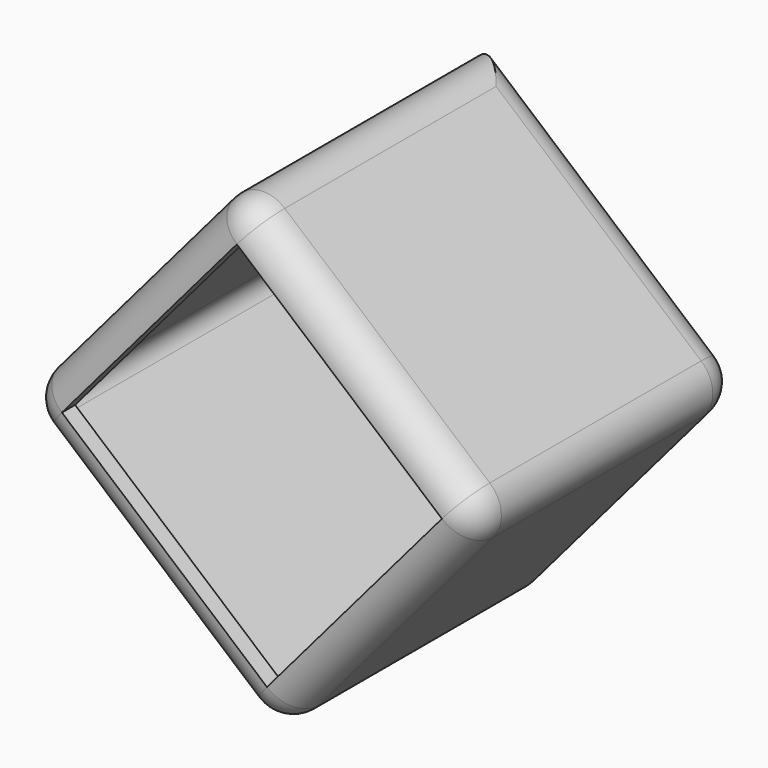
from build123d import *

# Parameters (mm, degrees)
F1_DEPTH = 50.8
F2_R     = 5.08
F3_T     = -2.54


# Not quite as in the source:
# - a shell that OpenCascade refuses in one call is made with other operations: the cavity is built on its own and cut out


with BuildPart() as f1:
    # F0 (on Front) → F1 (new body)
    with BuildSketch(Plane.XZ):
        Polygon((-36.388931796, -2.8822999448), (2.8822999448, -36.388931796), (36.388931796, 2.8822999448), (-2.8822999448, 36.388931796), align=None)
    extrude(amount=F1_DEPTH)

    # F2
    f2_edges = [f1.edges().sort_by_distance(p)[0] for p in [
        (36.388932, -25.4, 2.8823),
        (-2.8823, -25.4, 36.388932),
        (16.753316, 0, 19.635616),
        (16.753316, -50.8, 19.635616),
        (-19.635616, -50.8, 16.753316),
        (-16.753316, -50.8, -19.635616),
        (19.635616, -50.8, -16.753316),
        (2.8823, -25.4, -36.388932),
        (19.635616, 0, -16.753316),
        (-36.388932, -25.4, -2.8823),
        (-16.753316, 0, -19.635616),
    ]]
    fillet(f2_edges, radius=F2_R)

    # F3: a shell. OpenCascade refuses it in one call, so the cavity is built on its own and cut out:
    # the body offset inwards by the wall thickness, plus a prism from it out through each open face.
    f3_core = offset(f1.part, amount=F3_T, mode=Mode.PRIVATE)
    f3_exits = [f3_core.faces().sort_by_distance(p)[0] for p in [
        (0, -48.26, 0),
    ]]
    add(f3_core, mode=Mode.SUBTRACT)
    extrude(f3_exits, amount=-F3_T, mode=Mode.SUBTRACT)


solid = f1.part
